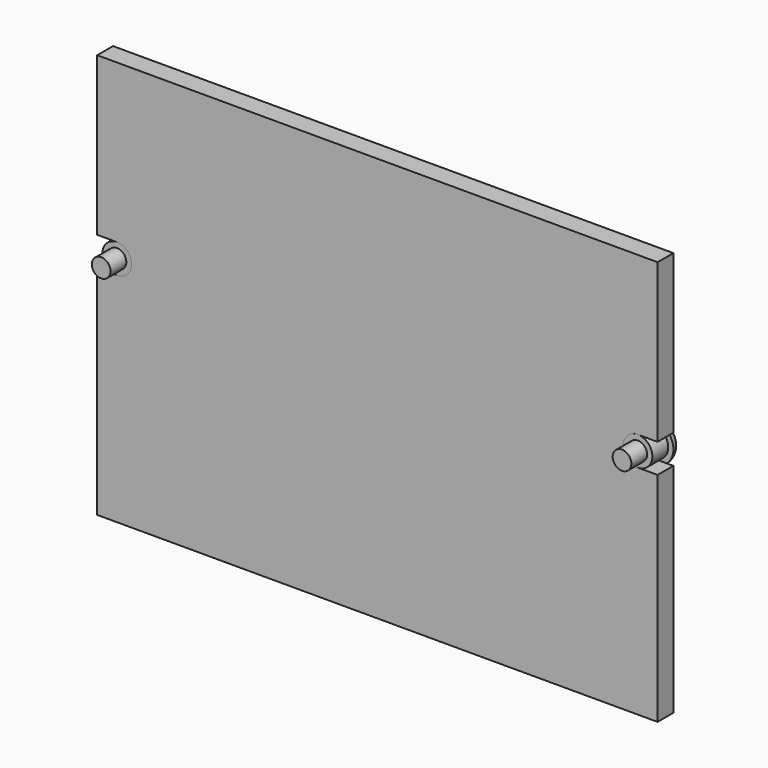
from build123d import *

# Parameters (mm, degrees)
F1_DEPTH  = 3.175
F3_DEPTH  = 1.5875
F4_R      = 1.58749
F4_2_R    = 1.58749
F6_DEPTH  = 0.79375
F8_R      = 2.3375
F9_DEPTH  = 3.175
F7_R      = 2.3375
F11_R     = 1.5
F12_DEPTH = 3.175
F10_R     = 1.5


# Not quite as in the source:
# - a fillet or chamfer is up to 0.001 mm smaller than in the source, because OpenCascade refuses the exact size


with BuildPart() as f1:
    # F0 (on Front) → F1 (new body)
    with BuildSketch(Plane.XZ):
        with BuildLine():
            Line((36.9228013605, 50.8562061697), (-53.0771986395, 50.8562061697))
            Line((-53.0771986395, 50.8562061697), (-53.0771986395, 25.4562061697))
            Line((-53.0771986395, 25.4562061697), (-49.9021986395, 25.4562061697))
            ThreePointArc((-49.9021986395, 25.4562061697), (-47.5646986395, 23.1187061697), (-49.9021986395, 20.7812061697))
            Line((-49.9021986395, 20.7812061697), (-53.0771986395, 20.7812061697))
            Line((-53.0771986395, 20.7812061697), (-53.0771986395, -14.1437938303))
            Line((-53.0771986395, -14.1437938303), (36.9228013605, -14.1437938303))
            Line((36.9228013605, -14.1437938303), (36.9228013605, 20.7812061697))
            Line((36.9228013605, 20.7812061697), (33.7478013605, 20.7812061697))
            ThreePointArc((33.7478013605, 20.7812061697), (31.4103013605, 23.1187061697), (33.7478013605, 25.4562061697))
            Line((33.7478013605, 25.4562061697), (36.9228013605, 25.4562061697))
            Line((36.9228013605, 25.4562061697), (36.9228013605, 50.8562061697))
        make_face()
    extrude(amount=F1_DEPTH)


with BuildPart() as f3:
    # F2 (on face) → F3 (new body)
    with BuildSketch(Plane(origin=(0, 0, 0), x_dir=(-1, 0, 0), z_dir=(0, 1, 0))):
        with BuildLine():
            Line((-33.7478013605, 25.4562061697), (-35.8964564631, 25.4562061697))
            ThreePointArc((-35.8964564631, 25.4562061697), (-36.9228013605, 23.1187061697), (-35.8964564631, 20.7812061697))
            Line((-35.8964564631, 20.7812061697), (-33.7478013605, 20.7812061697))
            ThreePointArc((-33.7478013605, 20.7812061697), (-31.4103013605, 23.1187061697), (-33.7478013605, 25.4562061697))
        make_face()
        with BuildLine():
            ThreePointArc((-35.8964564631, 20.7812061697), (-32.4713521744, 20.211593775), (-30.5728013605, 23.1187061697))
            ThreePointArc((-30.5728013605, 23.1187061697), (-32.4713521744, 26.0258185644), (-35.8964564631, 25.4562061697))
            Line((-35.8964564631, 25.4562061697), (-33.7478013605, 25.4562061697))
            ThreePointArc((-33.7478013605, 25.4562061697), (-31.4103013605, 23.1187061697), (-33.7478013605, 20.7812061697))
            Line((-33.7478013605, 20.7812061697), (-35.8964564631, 20.7812061697))
        make_face()
    extrude(amount=F3_DEPTH)

    # F4 (radius 1.5875 in the source; OpenCascade refuses exactly that, so slightly less here)
    f4_edges = [f3.edges().sort_by_distance(p)[0] for p in [
        (31.599146, 1.5875, 25.456206),
    ]]
    fillet(f4_edges, radius=F4_R)


with BuildPart() as f3b:
    # F2 (on face) → F3, piece 2 (new body)
    with BuildSketch(Plane(origin=(0, 0, 0), x_dir=(-1, 0, 0), z_dir=(0, 1, 0))):
        with BuildLine():
            ThreePointArc((53.0771986395, 23.1187061697), (52.8093110342, 24.3951553557), (52.0508537421, 25.4562061697))
            Line((52.0508537421, 25.4562061697), (49.9021986395, 25.4562061697))
            ThreePointArc((49.9021986395, 25.4562061697), (47.5646986395, 23.1187061697), (49.9021986395, 20.7812061697))
            Line((49.9021986395, 20.7812061697), (52.0508537421, 20.7812061697))
            ThreePointArc((52.0508537421, 20.7812061697), (52.8093110342, 21.8422569836), (53.0771986395, 23.1187061697))
        make_face()
        with BuildLine():
            Line((49.9021986395, 25.4562061697), (52.0508537421, 25.4562061697))
            ThreePointArc((52.0508537421, 25.4562061697), (46.7271986395, 23.1187061697), (52.0508537421, 20.7812061697))
            Line((52.0508537421, 20.7812061697), (49.9021986395, 20.7812061697))
            ThreePointArc((49.9021986395, 20.7812061697), (47.5646986395, 23.1187061697), (49.9021986395, 25.4562061697))
        make_face()
    extrude(amount=F3_DEPTH)

    # F4#2 (radius 1.5875 in the source; OpenCascade refuses exactly that, so slightly less here)
    f4_2_edges = [f3b.edges().sort_by_distance(p)[0] for p in [
        (-46.727199, 1.5875, 23.118706),
    ]]
    fillet(f4_2_edges, radius=F4_2_R)


with BuildPart() as f6_tool:
    # F5 (on face) → F6 (new body)
    with BuildSketch(Plane(origin=(0, 1.5875, 0), x_dir=(-1, 0, 0), z_dir=(0, 1, 0))):
        with BuildLine():
            Line((-33.5003139871, 23.3661935431), (-33.4987591805, 24.6865601146))
            ThreePointArc((-33.4987591805, 24.6865601146), (-33.7478013605, 24.7062161697), (-33.9968435405, 24.6865601146))
            Line((-33.9968435405, 24.6865601146), (-33.9952887339, 23.3661935431))
            Line((-33.9952887339, 23.3661935431), (-35.3156553054, 23.3677483496))
            ThreePointArc((-35.3156553054, 23.3677483496), (-35.3353113605, 23.1187061697), (-35.3156553054, 22.8696639897))
            Line((-35.3156553054, 22.8696639897), (-33.9952887339, 22.8712187962))
            Line((-33.9952887339, 22.8712187962), (-33.9968435405, 21.5508522247))
            ThreePointArc((-33.9968435405, 21.5508522247), (-33.7478013605, 21.5311961697), (-33.4987591805, 21.5508522247))
            Line((-33.4987591805, 21.5508522247), (-33.5003139871, 22.8712187962))
            Line((-33.5003139871, 22.8712187962), (-32.1799474155, 22.8696639897))
            ThreePointArc((-32.1799474155, 22.8696639897), (-32.1652130034, 22.9937978354), (-32.1602913605, 23.1187061697))
            ThreePointArc((-32.1602913605, 23.1187061697), (-32.1652130034, 23.243614504), (-32.1799474155, 23.3677483496))
            Line((-32.1799474155, 23.3677483496), (-33.5003139871, 23.3661935431))
        make_face()
        with BuildLine():
            Line((-33.4978013605, 25.4999561697), (-33.7478013605, 25.4999561697))
            Line((-33.7478013605, 25.4999561697), (-33.9978013605, 25.4999561697))
            Line((-33.9978013605, 25.4999561697), (-33.9968435405, 24.6865601146))
            ThreePointArc((-33.9968435405, 24.6865601146), (-33.7478013605, 24.7062161697), (-33.4987591805, 24.6865601146))
            Line((-33.4987591805, 24.6865601146), (-33.4978013605, 25.4999561697))
        make_face()
        with BuildLine():
            Line((-31.3665513605, 23.3687061697), (-32.1799474155, 23.3677483496))
            ThreePointArc((-32.1799474155, 23.3677483496), (-32.1652130034, 23.243614504), (-32.1602913605, 23.1187061697))
            ThreePointArc((-32.1602913605, 23.1187061697), (-32.1652130034, 22.9937978354), (-32.1799474155, 22.8696639897))
            Line((-32.1799474155, 22.8696639897), (-31.3665513605, 22.8687061697))
            Line((-31.3665513605, 22.8687061697), (-31.3665513605, 23.1187061697))
            Line((-31.3665513605, 23.1187061697), (-31.3665513605, 23.3687061697))
        make_face()
        with BuildLine():
            ThreePointArc((-33.4987591805, 21.5508522247), (-33.7478013605, 21.5311961697), (-33.9968435405, 21.5508522247))
            Line((-33.9968435405, 21.5508522247), (-33.9978013605, 20.7374561697))
            Line((-33.9978013605, 20.7374561697), (-33.7478013605, 20.7374561697))
            Line((-33.7478013605, 20.7374561697), (-33.4978013605, 20.7374561697))
            Line((-33.4978013605, 20.7374561697), (-33.4987591805, 21.5508522247))
        make_face()
        with BuildLine():
            ThreePointArc((-35.3156553054, 22.8696639897), (-35.3353113605, 23.1187061697), (-35.3156553054, 23.3677483496))
            Line((-35.3156553054, 23.3677483496), (-36.1290513605, 23.3687061697))
            Line((-36.1290513605, 23.3687061697), (-36.1290513605, 23.1187061697))
            Line((-36.1290513605, 23.1187061697), (-36.1290513605, 22.8687061697))
            Line((-36.1290513605, 22.8687061697), (-35.3156553054, 22.8696639897))
        make_face()
        Polygon((49.6521986395, 20.7374561697), (49.9021986395, 20.7374561697), (50.1521986395, 20.7374561697), (50.1496860129, 22.8712187962), (52.2834486395, 22.8687061697), (52.2834486395, 23.1187061697), (52.2834486395, 23.3687061697), (50.1496860129, 23.3661935431), (50.1521986395, 25.4999561697), (49.9021986395, 25.4999561697), (49.6521986395, 25.4999561697), (49.6547112661, 23.3661935431), (47.5209486395, 23.3687061697), (47.5209486395, 23.1187061697), (47.5209486395, 22.8687061697), (49.6547112661, 22.8712187962), align=None)
    extrude(amount=-F6_DEPTH)


with BuildPart() as f3_1:
    add(f3.part)

    # F6: cut by f6_tool
    add(f6_tool.part, mode=Mode.SUBTRACT)

    # F7 (on face) → F9, piece 2 (join, through all)
    with BuildSketch(Plane.XZ):
        with Locations((33.7478013605, 23.1187061697)):
            Circle(F7_R)
    extrude(amount=F9_DEPTH)

    # F10 (on face) → F12, piece 2 (join)
    with BuildSketch(Plane.XZ.offset(3.175)):
        with Locations((33.7478013605, 23.1187061697)):
            Circle(F10_R)
    extrude(amount=F12_DEPTH)


with BuildPart() as f3b_1:
    add(f3b.part)

    # F6: cut by f6_tool
    add(f6_tool.part, mode=Mode.SUBTRACT)

    # F8 (on face) → F9 (join, through all)
    with BuildSketch(Plane.XZ):
        with Locations((-49.9021986395, 23.1187061697)):
            Circle(F8_R)
    extrude(amount=F9_DEPTH)

    # F11 (on face) → F12 (join)
    with BuildSketch(Plane.XZ.offset(3.175)):
        with Locations((-49.9021986395, 23.1187061697)):
            Circle(F11_R)
    extrude(amount=F12_DEPTH)


solid = Compound([f1.part, f3_1.part, f3b_1.part])
